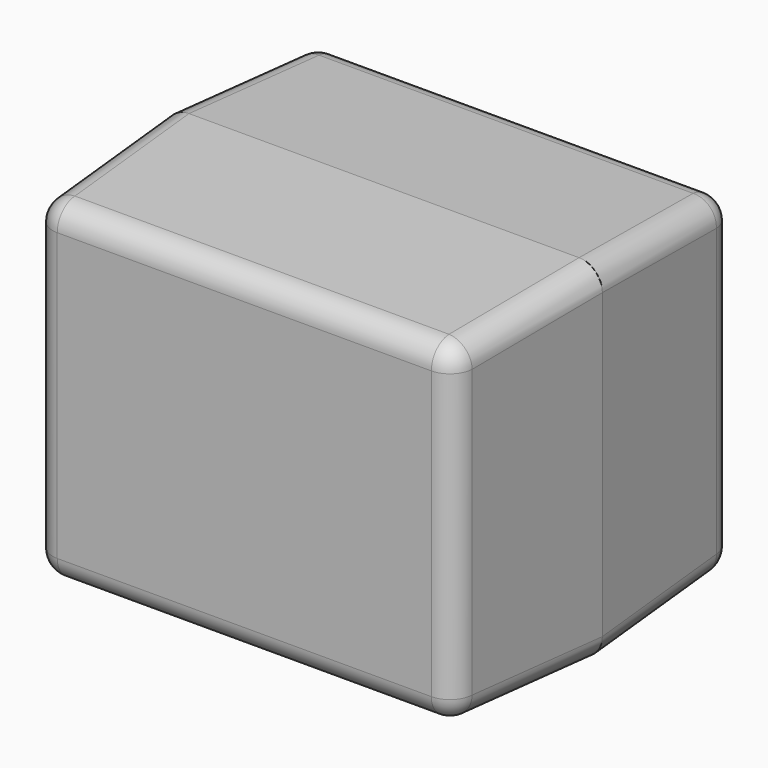
from build123d import *

# Parameters (mm, degrees)
F0_W     = 95.25
F0_H     = 76.2
F1_DEPTH = 38.1
F1_TAPER = 3
F2_R     = 5.08
F4_D     = 31.75
F4_DEPTH = 12.7
F4_TIP   = 9.5386623271


with BuildPart() as f1:
    # F0 (on Front) → F1 (new body, symmetric)
    with BuildSketch(Plane.XZ):
        with Locations((-1.951872288, -1.5614978304)):
            Rectangle(F0_W, F0_H)
    extrude(amount=F1_DEPTH, both=True, taper=F1_TAPER)

    # F2
    f2_edges = [f1.edges().sort_by_distance(p)[0] for p in [
        (43.676391, -38.1, -1.561498),
        (-1.951872, -38.1, 34.541766),
        (-47.580136, -38.1, -1.561498),
        (-1.951872, -38.1, -37.664761),
        (43.676391, 38.1, -1.561498),
        (-1.951872, 38.1, 34.541766),
        (-47.580136, 38.1, -1.561498),
        (-1.951872, 38.1, -37.664761),
        (44.67476, -19.05, 35.540134),
        (44.67476, -19.05, -38.66313),
        (44.67476, 19.05, 35.540134),
        (44.67476, 19.05, -38.66313),
        (-48.578504, -19.05, 35.540134),
        (-48.578504, -19.05, -38.66313),
        (-48.578504, 19.05, 35.540134),
        (-48.578504, 19.05, -38.66313),
    ]]
    fillet(f2_edges, radius=F2_R)

    # F4
    with Locations(Plane(origin=(0, 38.1, 0), x_dir=(-1, 0, 0), z_dir=(0, 1, 0))):
        with Locations((0, 0)):
            Hole(F4_D / 2, depth=F4_DEPTH)
            with Locations((0, 0, -(F4_DEPTH + F4_TIP / 2))):  # 118° drill point
                Cone(0, F4_D / 2, F4_TIP, mode=Mode.SUBTRACT)


solid = f1.part
